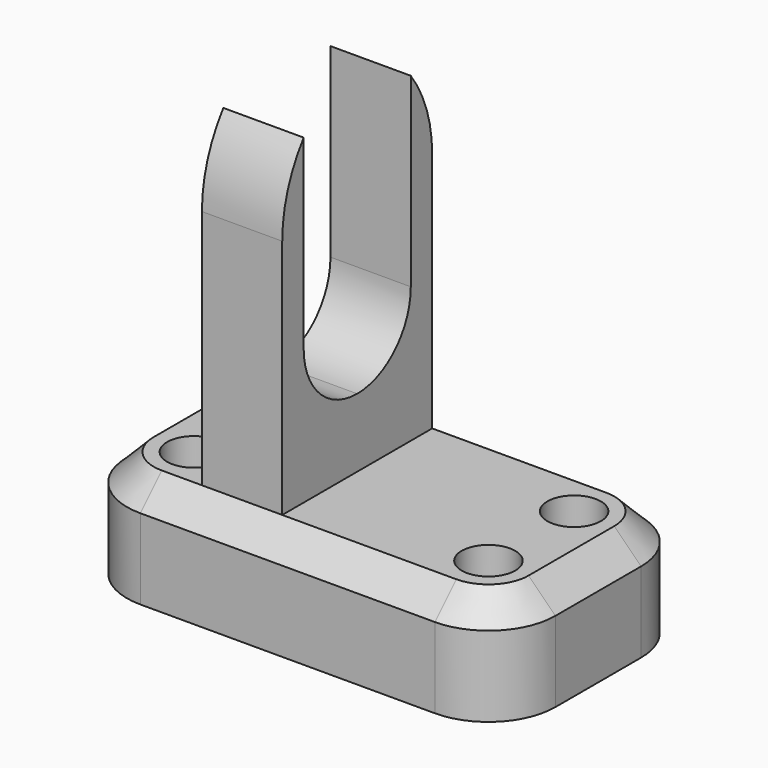
from build123d import *

# Parameters (mm, degrees)
F0_R        = 6.35
F1_DEPTH    = 25.4
F2_SIZE     = 6.35
F3_W        = 19.05
F3_H        = 44.45
F4_DEPTH    = 76.2
F6_DEPTH    = 19.05
F8_DEPTH    = 25.4
F9_T1_DEPTH = 114.3


# Not quite as in the source:
# - a fillet or chamfer that OpenCascade refuses, or shapes differently, is made with other operations: its cross-section is extruded or revolved along the edge and cut away or added


with BuildPart() as f1:
    # F0 (on Top) → F1 (new body)
    with BuildSketch(Plane.XY):
        with BuildLine():
            Line((-4.9749455661, 42.822749579), (-74.8249455661, 42.822749579))
            ThreePointArc((-74.8249455661, 42.822749579), (-86.0502657174, 38.1730697303), (-90.6999455661, 26.947749579))
            Line((-90.6999455661, 26.947749579), (-90.6999455661, 1.547749579))
            ThreePointArc((-90.6999455661, 1.547749579), (-86.0502657174, -9.6775705724), (-74.8249455661, -14.327250421))
            Line((-74.8249455661, -14.327250421), (-4.9749455661, -14.327250421))
            ThreePointArc((-4.9749455661, -14.327250421), (6.2503745853, -9.6775705724), (10.9000544339, 1.547749579))
            Line((10.9000544339, 1.547749579), (10.9000544339, 26.947749579))
            ThreePointArc((10.9000544339, 26.947749579), (6.2503745853, 38.1730697303), (-4.9749455661, 42.822749579))
        make_face()
        with Locations((-74.8249455661, 1.547749579)):
            Circle(F0_R, mode=Mode.SUBTRACT)
        with Locations((-4.9749455661, 1.547749579)):
            Circle(F0_R, mode=Mode.SUBTRACT)
        with Locations((-74.8249455661, 26.947749579)):
            Circle(F0_R, mode=Mode.SUBTRACT)
        with Locations((-4.9749455661, 26.947749579)):
            Circle(F0_R, mode=Mode.SUBTRACT)
    extrude(amount=F1_DEPTH)

    # F2
    f2_edges = [f1.edges().sort_by_distance(p)[0] for p in [
        (6.250375, -9.677571, 25.4),
        (10.900054, 14.24775, 25.4),
        (6.250375, 38.17307, 25.4),
        (-39.899946, 42.82275, 25.4),
        (-86.050266, 38.17307, 25.4),
        (-90.699946, 14.24775, 25.4),
        (-86.050266, -9.677571, 25.4),
        (-39.899946, -14.32725, 25.4),
    ]]
    chamfer(f2_edges, length=F2_SIZE)

    # F3 (on face) → F4 (join)
    with BuildSketch(Plane.XY.offset(25.4)):
        with Locations((-55.7749455661, 14.247749579)):
            Rectangle(F3_W, F3_H)
    extrude(amount=F4_DEPTH)

    # F5 (on face) → F6 (cut, through all)
    with BuildSketch(Plane.YZ.offset(-46.2499455661)):
        with BuildLine():
            ThreePointArc((14.247749579, 41.6659471005), (25.4730697303, 46.3156269492), (30.122749579, 57.5409471005))
            ThreePointArc((30.122749579, 57.5409471005), (3.0224294276, 68.7662672519), (14.247749579, 41.6659471005))
        make_face()
    extrude(amount=-F6_DEPTH, mode=Mode.SUBTRACT)

    # F7 (on face) → F8 (cut)
    with BuildSketch(Plane.YZ.offset(-46.2499455661)):
        with BuildLine():
            ThreePointArc((-1.627250421, 57.5409471005), (14.247749579, 73.4159471005), (30.122749579, 57.5409471005))
            Line((30.122749579, 57.5409471005), (30.122749579, 101.6))
            Line((30.122749579, 101.6), (-1.627250421, 101.6))
            Line((-1.627250421, 101.6), (-1.627250421, 57.5409471005))
        make_face()
    extrude(amount=-F8_DEPTH, mode=Mode.SUBTRACT)

    # F9: fillet of radius 31.75 on 2 edges, made by hand

    # F9_s2 → F9_t1 (cut)
    with BuildSketch(Plane.YZ.offset(-112.9249455661)):
        with BuildLine():
            ThreePointArc((-7.977250421, 82.55), (-6.3479451342, 92.590231571), (-1.627250421, 101.6))
            Line((-1.627250421, 101.6), (-7.977250421, 101.6))
            Line((-7.977250421, 101.6), (-7.977250421, 82.55))
        make_face()
        with BuildLine():
            ThreePointArc((36.472749579, 82.55), (34.8434442921, 92.590231571), (30.122749579, 101.6))
            Line((30.122749579, 101.6), (36.472749579, 101.6))
            Line((36.472749579, 101.6), (36.472749579, 82.55))
        make_face()
    extrude(amount=F9_T1_DEPTH, mode=Mode.SUBTRACT)


solid = f1.part
